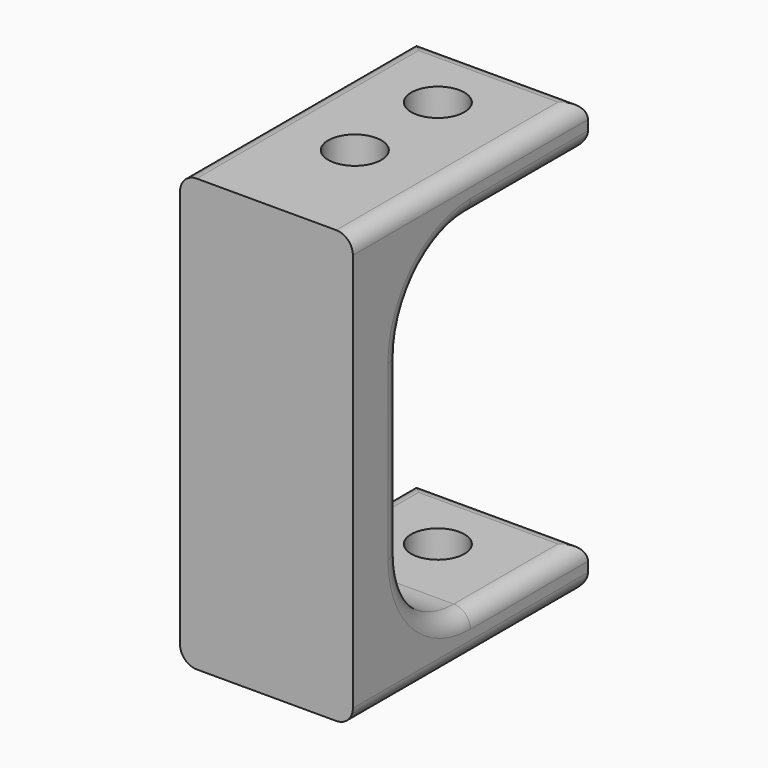
from build123d import *

# Parameters (mm, degrees)
F1_DEPTH     = 10
F2_R         = 1.538196108
F3_DEPTH     = 25
F4_T4_DEPTH  = 10
F4_S5_R      = 1.538196108
F4_T6_DEPTH  = 8
F4_T10_DEPTH = 10
F4_S11_R     = 1.538196108
F4_T12_DEPTH = 8
F5_R         = 0.9656854249


# Not quite as in the source:
# - a fillet or chamfer that OpenCascade refuses, or shapes differently, is made with other operations: its cross-section is extruded or revolved along the edge and cut away or added


with BuildPart() as f1:
    # F0 (on Right) → F1 (new body)
    with BuildSketch(Plane.YZ):
        Polygon((17, 0), (0, 0), (0, -25), (17, -25), (17, -22.5), (3.5, -22.5), (3.5, -2.5), (17, -2.5), align=None)
    extrude(amount=F1_DEPTH)

    # F2 (on face) → F3 (cut)
    with BuildSketch(Plane(origin=(0, 0, -25), x_dir=(1, 0, 0), z_dir=(0, 0, -1))):
        with Locations((4.8035508953, -6.6337394528)):
            Circle(F2_R)
        with Locations((4.8077256637, -12.6337380004)):
            Circle(F2_R)
    extrude(amount=-F3_DEPTH, mode=Mode.SUBTRACT)

    # F4: fillet of radius 5 on 2 edges, made by hand


with BuildPart() as f4_tool2:
    # F4_s3 → F4_t4 (new body)
    with BuildSketch(Plane.YZ):
        with BuildLine():
            ThreePointArc((8.5, -2.5), (4.9644660941, -3.9644660941), (3.5, -7.5))
            Line((3.5, -7.5), (3.5, -2.5))
            Line((3.5, -2.5), (8.5, -2.5))
        make_face()
    extrude(amount=F4_T4_DEPTH)

    # F4_s5 → F4_t6 (cut, symmetric)
    with BuildSketch(Plane.XY.offset(-5)):
        with Locations((4.8035508953, 6.6337394528)):
            Circle(F4_S5_R)
    extrude(amount=F4_T6_DEPTH, both=True, mode=Mode.SUBTRACT)


with BuildPart() as f1_1:
    add(f1.part)

    # F4_t1: union F4_tool2
    add(f4_tool2.part)


with BuildPart() as f4_tool8:
    # F4_s9 → F4_t10 (new body)
    with BuildSketch(Plane.YZ):
        with BuildLine():
            ThreePointArc((8.5, -22.5), (4.9644660941, -21.0355339059), (3.5, -17.5))
            Line((3.5, -17.5), (3.5, -22.5))
            Line((3.5, -22.5), (8.5, -22.5))
        make_face()
    extrude(amount=F4_T10_DEPTH)

    # F4_s11 → F4_t12 (cut, symmetric)
    with BuildSketch(Plane.XY.offset(-20)):
        with Locations((4.8035508953, 6.6337394528)):
            Circle(F4_S11_R)
    extrude(amount=F4_T12_DEPTH, both=True, mode=Mode.SUBTRACT)


with BuildPart() as f1_2:
    add(f1_1.part)

    # F4_t7: union F4_tool8
    add(f4_tool8.part)

    # F5
    f5_edges = [f1_2.edges().sort_by_distance(p)[0] for p in [
        (5, 17, -22.5),
        (5, 17, -25),
        (5, 17, 0),
        (5, 17, -2.5),
        (0, 8.5, 0),
        (10, 8.5, 0),
        (10, 8.5, -25),
        (0, 8.5, -25),
        (10, 4.964466, -3.964466),
        (0, 4.964466, -3.964466),
        (0, 3.5, -12.5),
    ]]
    fillet(f5_edges, radius=F5_R)


solid = f1_2.part
